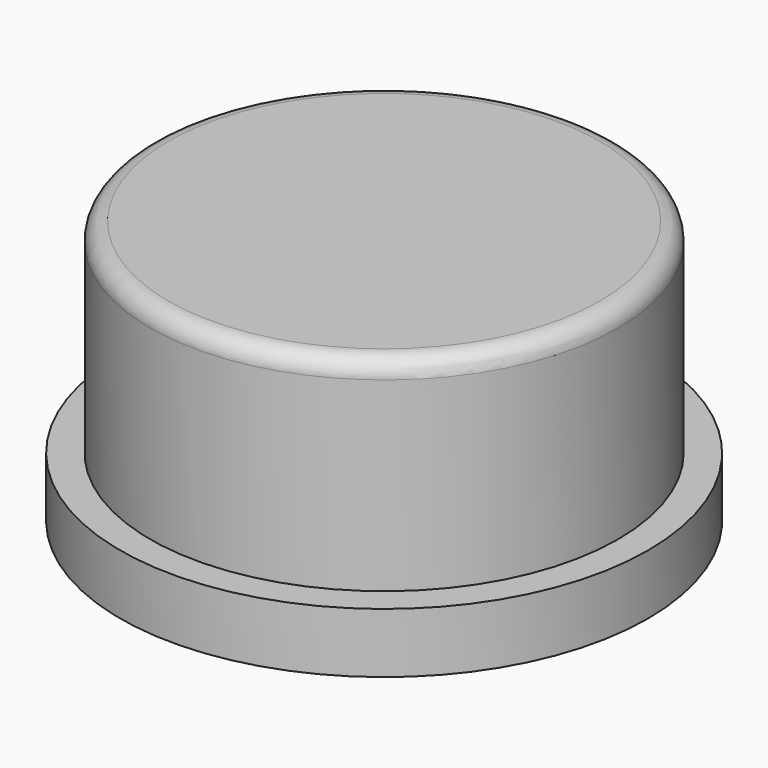
from build123d import *

# Parameters (mm, degrees)
F0_R     = 4.4
F0_R_2   = 3.9
F1_DEPTH = 1
F2_DEPTH = 4.4
F3_R     = 0.3


# Not quite as in the source:
# - a feature names something its author has since deleted; it is built from what else it names


with BuildPart() as f1:
    # F0 (on Top) → F1 (new body)
    with BuildSketch(Plane.XY):
        with Locations((-17.6290911883, 6.9914618582)):
            Circle(F0_R)
        with Locations((-17.6290911883, 6.9914618582)):
            Circle(F0_R_2, mode=Mode.SUBTRACT)
        with Locations((-17.6290911883, 6.9914618582)):
            Circle(F0_R_2)
    extrude(amount=F1_DEPTH)

    # F0 (on Top) → F2 (join)
    with BuildSketch(Plane.XY):
        with Locations((-17.6290911883, 6.9914618582)):
            Circle(F0_R_2)
    extrude(amount=F2_DEPTH)

    # F3
    f3_edges = [f1.edges().sort_by_distance(p)[0] for p in [
        (-21.529091, 6.991462, 4.4),
    ]]
    fillet(f3_edges, radius=F3_R)


solid = f1.part
